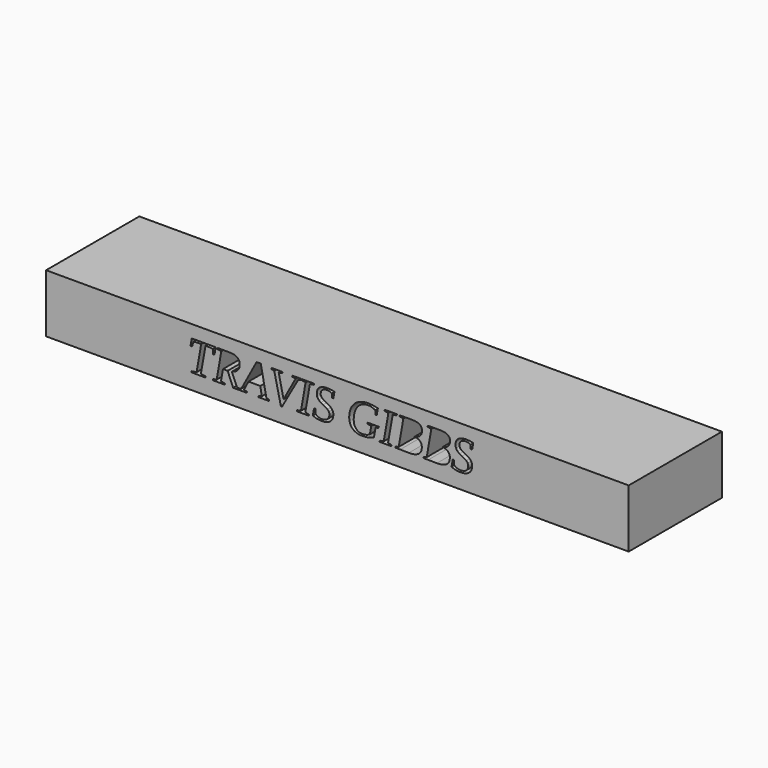
from build123d import *

# Parameters (mm, degrees)
F0_W     = 127
F0_H     = 12.7
F1_DEPTH = 25.4


with BuildPart() as f1:
    # F0 (on Front) → F1 (new body)
    with BuildSketch(Plane.XZ):
        with Locations((-1.1512227356, 52.6019901231)):
            Rectangle(F0_W, F0_H)
        with BuildLine():
            Line((-29.9385481048, 49.6464967728), (-32.9583853923, 49.6464967728))
            Line((-32.9583853923, 49.6464967728), (-32.9099805547, 49.9056968709))
            Line((-32.9099805547, 49.9056968709), (-31.8513199131, 50.0368583663))
            Line((-31.8513199131, 50.0368583663), (-30.8410641091, 55.7704894519))
            Line((-30.8410641091, 55.7704894519), (-31.0893340825, 55.7704894519))
            add(Edge.make_bspline(
                [(-31.0893340825, 55.7704894519), (-32.0605537272, 55.7704894519), (-32.5243033003, 55.6721183303)],
                knots=[0, 0, 0, 1, 1, 1], degree=2))
            Line((-32.5243033003, 55.6721183303), (-32.8365925751, 54.6524938481))
            Line((-32.8365925751, 54.6524938481), (-33.1629348673, 54.6524938481))
            Line((-33.1629348673, 54.6524938481), (-32.8896817518, 56.1905185265))
            Line((-32.8896817518, 56.1905185265), (-27.6682050769, 56.1905185265))
            Line((-27.6682050769, 56.1905185265), (-27.9414581924, 54.6524938481))
            Line((-27.9414581924, 54.6524938481), (-28.2740462701, 54.6524938481))
            Line((-28.2740462701, 54.6524938481), (-28.2256414325, 55.6721183303))
            add(Edge.make_bspline(
                [(-28.2256414325, 55.6721183303), (-28.6644078636, 55.7611207736), (-29.6590492039, 55.7611207736)],
                knots=[0, 0, 0, 1, 1, 1], degree=2))
            Line((-29.6590492039, 55.7611207736), (-29.8995119455, 55.7611207736))
            Line((-29.8995119455, 55.7611207736), (-30.9082063031, 50.0368583663))
            Line((-30.9082063031, 50.0368583663), (-29.8885818209, 49.9056968709))
            Line((-29.8885818209, 49.9056968709), (-29.9385481048, 49.6464967728))
        make_face(mode=Mode.SUBTRACT)
        with BuildLine():
            Line((-25.0730812032, 52.5164352083), (-26.0927056855, 52.5164352083))
            Line((-26.0927056855, 52.5164352083), (-26.533033563, 50.0368583663))
            Line((-26.533033563, 50.0368583663), (-25.6586235935, 49.9056968709))
            Line((-25.6586235935, 49.9056968709), (-25.7085898775, 49.6464967728))
            Line((-25.7085898775, 49.6464967728), (-28.3130824294, 49.6464967728))
            Line((-28.3130824294, 49.6464967728), (-28.2646775918, 49.9056968709))
            Line((-28.2646775918, 49.9056968709), (-27.4745857265, 50.0368583663))
            Line((-27.4745857265, 50.0368583663), (-26.4549612443, 55.8048412721))
            Line((-26.4549612443, 55.8048412721), (-27.2747205907, 55.9313184284))
            Line((-27.2747205907, 55.9313184284), (-27.2247543067, 56.1905185265))
            Line((-27.2247543067, 56.1905185265), (-24.629630433, 56.1905185265))
            add(Edge.make_bspline(
                [(-24.629630433, 56.1905185265), (-23.5616011131, 56.1905185265), (-23.0002611416, 55.7853231924)],
                knots=[0, 0, 0, 1, 1, 1], degree=2))
            add(Edge.make_bspline(
                [(-23.0002611416, 55.7853231924), (-22.4389211702, 55.3801278584), (-22.4389211702, 54.6040890105)],
                knots=[0, 0, 0, 1, 1, 1], degree=2))
            add(Edge.make_bspline(
                [(-22.4389211702, 54.6040890105), (-22.4389211702, 53.0629414392), (-24.1471435034, 52.6522810429)],
                knots=[0, 0, 0, 1, 1, 1], degree=2))
            Line((-24.1471435034, 52.6522810429), (-23.0385165778, 50.0368583663))
            Line((-23.0385165778, 50.0368583663), (-22.5105122318, 49.94023012))
            Line((-22.5105122318, 49.94023012), (-22.1078945389, 50.0368583663))
            Line((-22.1078945389, 50.0368583663), (-18.7788908693, 56.2436077032))
            Line((-18.7788908693, 56.2436077032), (-17.8482688304, 56.2436077032))
            Line((-17.8482688304, 56.2436077032), (-16.6272177658, 50.0368583663))
            Line((-16.6272177658, 50.0368583663), (-16.01825368, 49.9056968709))
            Line((-16.01825368, 49.9056968709), (-16.0713428567, 49.6464967728))
            Line((-16.0713428567, 49.6464967728), (-18.3885292758, 49.6464967728))
            Line((-18.3885292758, 49.6464967728), (-18.3354400991, 49.9056968709))
            Line((-18.3354400991, 49.9056968709), (-17.6374735699, 50.0368583663))
            Line((-17.6374735699, 50.0368583663), (-17.9497628447, 51.9246470325))
            Line((-17.9497628447, 51.9246470325), (-20.5261493619, 51.9246470325))
            Line((-20.5261493619, 51.9246470325), (-21.5270364877, 50.0368583663))
            Line((-21.5270364877, 50.0368583663), (-20.8681061178, 49.9056968709))
            Line((-20.8681061178, 49.9056968709), (-20.9165109554, 49.6464967728))
            Line((-20.9165109554, 49.6464967728), (-22.3702175297, 49.6464967728))
            Line((-22.3702175297, 49.6464967728), (-22.7028056074, 49.6464967728))
            Line((-22.7028056074, 49.6464967728), (-23.8738903879, 49.6464967728))
            Line((-23.8738903879, 49.6464967728), (-25.0730812032, 52.5164352083))
        make_face(mode=Mode.SUBTRACT)
        Polygon((-10.9529216425, 56.1905185265), (-8.9870606575, 56.1905185265), (-9.0354654951, 55.9313184284), (-9.6756585085, 55.8048412721), (-13.221703224, 49.4950364745), (-13.4715346438, 49.4950364745), (-14.9111882007, 55.8048412721), (-15.5310824112, 55.9313184284), (-15.4811161273, 56.1905185265), (-13.0764887112, 56.1905185265), (-13.1248935488, 55.9313184284), (-13.9493372343, 55.8048412721), (-12.8859922536, 51.0268153674), (-10.2658852379, 55.8048412721), (-11.0075722655, 55.9313184284), align=None, mode=Mode.SUBTRACT)
        Polygon((-7.1383081506, 55.8048412721), (-8.1485639546, 50.0368583663), (-7.3381732865, 49.9056968709), (-7.3772094458, 49.6464967728), (-9.9879477833, 49.6464967728), (-9.9489116239, 49.9056968709), (-9.0901161182, 50.0368583663), (-8.0798603142, 55.8048412721), (-8.8902509823, 55.9313184284), (-8.851214823, 56.1905185265), (-6.2311078073, 56.1905185265), (-6.2701439666, 55.9313184284), align=None, mode=Mode.SUBTRACT)
        with BuildLine():
            Line((-6.5043609227, 50.0025065461), (-6.2498451637, 51.4562131203))
            Line((-6.2498451637, 51.4562131203), (-5.9328715498, 51.4562131203))
            Line((-5.9328715498, 51.4562131203), (-5.9281872107, 50.5255910814))
            add(Edge.make_bspline(
                [(-5.9281872107, 50.5255910814), (-5.7673582342, 50.2804440006), (-5.3793388102, 50.1125885154)],
                knots=[0, 0, 0, 1, 1, 1], degree=2))
            add(Edge.make_bspline(
                [(-5.3793388102, 50.1125885154), (-4.9913193862, 49.9447330302), (-4.5572372942, 49.9447330302)],
                knots=[0, 0, 0, 1, 1, 1], degree=2))
            add(Edge.make_bspline(
                [(-4.5572372942, 49.9447330302), (-3.7577767507, 49.9447330302), (-3.3252561051, 50.3226030527)],
                knots=[0, 0, 0, 1, 1, 1], degree=2))
            add(Edge.make_bspline(
                [(-3.3252561051, 50.3226030527), (-2.8927354595, 50.7004730753), (-2.8927354595, 51.3781408016)],
                knots=[0, 0, 0, 1, 1, 1], degree=2))
            add(Edge.make_bspline(
                [(-2.8927354595, 51.3781408016), (-2.8927354595, 51.6420252388), (-3.0098439375, 51.8372060356)],
                knots=[0, 0, 0, 1, 1, 1], degree=2))
            add(Edge.make_bspline(
                [(-3.0098439375, 51.8372060356), (-3.1269524156, 52.0323868324), (-3.3221332124, 52.1885314698)],
                knots=[0, 0, 0, 1, 1, 1], degree=2))
            add(Edge.make_bspline(
                [(-3.3221332124, 52.1885314698), (-3.5173140091, 52.3446761072), (-3.7640225362, 52.4766183258)],
                knots=[0, 0, 0, 1, 1, 1], degree=2))
            add(Edge.make_bspline(
                [(-3.7640225362, 52.4766183258), (-4.0107310633, 52.6085605444), (-4.2691504382, 52.7428449326)],
                knots=[0, 0, 0, 1, 1, 1], degree=2))
            add(Edge.make_bspline(
                [(-4.2691504382, 52.7428449326), (-4.5275698131, 52.8771293207), (-4.7742783402, 53.0309317886)],
                knots=[0, 0, 0, 1, 1, 1], degree=2))
            add(Edge.make_bspline(
                [(-4.7742783402, 53.0309317886), (-5.0209868673, 53.1847342564), (-5.2161676641, 53.3869415619)],
                knots=[0, 0, 0, 1, 1, 1], degree=2))
            add(Edge.make_bspline(
                [(-5.2161676641, 53.3869415619), (-5.4113484609, 53.5891488673), (-5.5284569389, 53.8530333045)],
                knots=[0, 0, 0, 1, 1, 1], degree=2))
            add(Edge.make_bspline(
                [(-5.5284569389, 53.8530333045), (-5.645565417, 54.1169177417), (-5.645565417, 54.472927515)],
                knots=[0, 0, 0, 1, 1, 1], degree=2))
            add(Edge.make_bspline(
                [(-5.645565417, 54.472927515), (-5.645565417, 55.341091699), (-5.0553386876, 55.8024991026)],
                knots=[0, 0, 0, 1, 1, 1], degree=2))
            add(Edge.make_bspline(
                [(-5.0553386876, 55.8024991026), (-4.4651119582, 56.2639065061), (-3.3674151572, 56.2639065061)],
                knots=[0, 0, 0, 1, 1, 1], degree=2))
            add(Edge.make_bspline(
                [(-3.3674151572, 56.2639065061), (-2.5273570079, 56.2639065061), (-1.7856699803, 56.0780943876)],
                knots=[0, 0, 0, 1, 1, 1], degree=2))
            Line((-1.7856699803, 56.0780943876), (-2.0245712755, 54.7165131494))
            Line((-2.0245712755, 54.7165131494), (-2.3415448894, 54.7165131494))
            Line((-2.3415448894, 54.7165131494), (-2.3665280314, 55.5503255131))
            add(Edge.make_bspline(
                [(-2.3665280314, 55.5503255131), (-2.5226726688, 55.6783641158), (-2.8006101234, 55.7658051128)],
                knots=[0, 0, 0, 1, 1, 1], degree=2))
            add(Edge.make_bspline(
                [(-2.8006101234, 55.7658051128), (-3.078547578, 55.8532461097), (-3.4392416904, 55.8532461097)],
                knots=[0, 0, 0, 1, 1, 1], degree=2))
            add(Edge.make_bspline(
                [(-3.4392416904, 55.8532461097), (-4.088803382, 55.8532461097), (-4.4401288162, 55.5362724958)],
                knots=[0, 0, 0, 1, 1, 1], degree=2))
            add(Edge.make_bspline(
                [(-4.4401288162, 55.5362724958), (-4.7914542504, 55.2192988818), (-4.7914542504, 54.6478095089)],
                knots=[0, 0, 0, 1, 1, 1], degree=2))
            add(Edge.make_bspline(
                [(-4.7914542504, 54.6478095089), (-4.7914542504, 54.3402045732), (-4.5720710348, 54.0864695374)],
                knots=[0, 0, 0, 1, 1, 1], degree=2))
            add(Edge.make_bspline(
                [(-4.5720710348, 54.0864695374), (-4.3526878192, 53.8327345017), (-3.9186057272, 53.6141320093)],
                knots=[0, 0, 0, 1, 1, 1], degree=2))
            add(Edge.make_bspline(
                [(-3.9186057272, 53.6141320093), (-3.2549910183, 53.2674909142), (-2.9622198231, 53.087143858)],
                knots=[0, 0, 0, 1, 1, 1], degree=2))
            add(Edge.make_bspline(
                [(-2.9622198231, 53.087143858), (-2.669448628, 52.9067968018), (-2.4719256617, 52.7014666036)],
                knots=[0, 0, 0, 1, 1, 1], degree=2))
            add(Edge.make_bspline(
                [(-2.4719256617, 52.7014666036), (-2.2744026953, 52.4961364055), (-2.1541713245, 52.2330326914)],
                knots=[0, 0, 0, 1, 1, 1], degree=2))
            add(Edge.make_bspline(
                [(-2.1541713245, 52.2330326914), (-2.0339399537, 51.9699289774), (-2.0339399537, 51.6279722215)],
                knots=[0, 0, 0, 1, 1, 1], degree=2))
            add(Edge.make_bspline(
                [(-2.0339399537, 51.6279722215), (-2.0339399537, 50.6224007566), (-2.690528154, 50.0852632039)],
                knots=[0, 0, 0, 1, 1, 1], degree=2))
            add(Edge.make_bspline(
                [(-2.690528154, 50.0852632039), (-3.3471163543, 49.5481256512), (-4.5869047754, 49.5481256512)],
                knots=[0, 0, 0, 1, 1, 1], degree=2))
            add(Edge.make_bspline(
                [(-4.5869047754, 49.5481256512), (-5.2021146467, 49.5481256512), (-5.6924088082, 49.6730413611)],
                knots=[0, 0, 0, 1, 1, 1], degree=2))
            add(Edge.make_bspline(
                [(-5.6924088082, 49.6730413611), (-6.1827029697, 49.7979570711), (-6.5043609227, 50.0025065461)],
                knots=[0, 0, 0, 1, 1, 1], degree=2))
        make_face(mode=Mode.SUBTRACT)
        with BuildLine():
            add(Edge.make_bspline(
                [(5.4703713201, 49.6714799148), (4.8754602515, 49.5590557758), (4.2399515773, 49.5590557758)],
                knots=[0, 0, 0, 1, 1, 1], degree=2))
            add(Edge.make_bspline(
                [(4.2399515773, 49.5590557758), (2.9080378202, 49.5590557758), (2.1663507925, 50.2593644746)],
                knots=[0, 0, 0, 1, 1, 1], degree=2))
            add(Edge.make_bspline(
                [(2.1663507925, 50.2593644746), (1.4246637648, 50.9596731734), (1.4246637648, 52.197900148)],
                knots=[0, 0, 0, 1, 1, 1], degree=2))
            add(Edge.make_bspline(
                [(1.4246637648, 52.197900148), (1.4246637648, 53.4236355517), (1.9321338364, 54.3456696355)],
                knots=[0, 0, 0, 1, 1, 1], degree=2))
            add(Edge.make_bspline(
                [(1.9321338364, 54.3456696355), (2.439603908, 55.2677037194), (3.3671030542, 55.7658051128)],
                knots=[0, 0, 0, 1, 1, 1], degree=2))
            add(Edge.make_bspline(
                [(3.3671030542, 55.7658051128), (4.2946022004, 56.2639065061), (5.4937930157, 56.2639065061)],
                knots=[0, 0, 0, 1, 1, 1], degree=2))
            add(Edge.make_bspline(
                [(5.4937930157, 56.2639065061), (6.6211572978, 56.2639065061), (7.6751336003, 55.9703545878)],
                knots=[0, 0, 0, 1, 1, 1], degree=2))
            Line((7.6751336003, 55.9703545878), (7.4268636268, 54.5650528511))
            Line((7.4268636268, 54.5650528511), (7.1005213346, 54.5650528511))
            Line((7.1005213346, 54.5650528511), (7.114574352, 55.3754435192))
            add(Edge.make_bspline(
                [(7.114574352, 55.3754435192), (6.4946801415, 55.8735449126), (5.4656869809, 55.8735449126)],
                knots=[0, 0, 0, 1, 1, 1], degree=2))
            add(Edge.make_bspline(
                [(5.4656869809, 55.8735449126), (4.6022071361, 55.8735449126), (3.8995562677, 55.4074531699)],
                knots=[0, 0, 0, 1, 1, 1], degree=2))
            add(Edge.make_bspline(
                [(3.8995562677, 55.4074531699), (3.1969053994, 54.9413614273), (2.8010787436, 54.0825659215)],
                knots=[0, 0, 0, 1, 1, 1], degree=2))
            add(Edge.make_bspline(
                [(2.8010787436, 54.0825659215), (2.4052520878, 53.2237704158), (2.4052520878, 52.1010904728)],
                knots=[0, 0, 0, 1, 1, 1], degree=2))
            add(Edge.make_bspline(
                [(2.4052520878, 52.1010904728), (2.4052520878, 51.0861503297), (2.9056956506, 50.5177838495)],
                knots=[0, 0, 0, 1, 1, 1], degree=2))
            add(Edge.make_bspline(
                [(2.9056956506, 50.5177838495), (3.4061392135, 49.9494173693), (4.3039708786, 49.9494173693)],
                knots=[0, 0, 0, 1, 1, 1], degree=2))
            add(Edge.make_bspline(
                [(4.3039708786, 49.9494173693), (4.7380529706, 49.9494173693), (5.1776001249, 50.0735523561)],
                knots=[0, 0, 0, 1, 1, 1], degree=2))
            add(Edge.make_bspline(
                [(5.1776001249, 50.0735523561), (5.6171472792, 50.1976873428), (5.9231907685, 50.3928681396)],
                knots=[0, 0, 0, 1, 1, 1], degree=2))
            Line((5.9231907685, 50.3928681396), (6.2307957042, 52.1151434902))
            Line((6.2307957042, 52.1151434902), (5.415720697, 52.2431820929))
            Line((5.415720697, 52.2431820929), (5.4610026418, 52.5055050837))
            Line((5.4610026418, 52.5055050837), (7.8749987361, 52.5055050837))
            Line((7.8749987361, 52.5055050837), (7.8312782377, 52.2431820929))
            Line((7.8312782377, 52.2431820929), (7.1676635287, 52.1151434902))
            Line((7.1676635287, 52.1151434902), (6.8022850772, 50.0665258474))
            add(Edge.make_bspline(
                [(6.8022850772, 50.0665258474), (6.0652823886, 49.7839040537), (5.4703713201, 49.6714799148)],
                knots=[0, 0, 0, 1, 1, 1], degree=2))
        make_face(mode=Mode.SUBTRACT)
        Polygon((10.9010818091, 55.8048412721), (9.8908260051, 50.0368583663), (10.7012166732, 49.9056968709), (10.6621805139, 49.6464967728), (8.0514421764, 49.6464967728), (8.0904783358, 49.9056968709), (8.9492738415, 50.0368583663), (9.9595296455, 55.8048412721), (9.1491389774, 55.9313184284), (9.1881751367, 56.1905185265), (11.8082821524, 56.1905185265), (11.7692459931, 55.9313184284), align=None, mode=Mode.SUBTRACT)
        with BuildLine():
            Line((12.5499691801, 49.6464967728), (11.510045895, 49.6464967728))
            Line((11.510045895, 49.6464967728), (11.560012179, 49.9056968709))
            Line((11.560012179, 49.9056968709), (12.2080124242, 50.0368583663))
            Line((12.2080124242, 50.0368583663), (13.2276369065, 55.8048412721))
            Line((13.2276369065, 55.8048412721), (12.4078775601, 55.9313184284))
            Line((12.4078775601, 55.9313184284), (12.4578438441, 56.1905185265))
            Line((12.4578438441, 56.1905185265), (15.1466545002, 56.1905185265))
            add(Edge.make_bspline(
                [(15.1466545002, 56.1905185265), (17.3030119428, 56.1905185265), (17.3030119428, 54.8133228246)],
                knots=[0, 0, 0, 1, 1, 1], degree=2))
            add(Edge.make_bspline(
                [(17.3030119428, 54.8133228246), (17.3030119428, 54.12628642), (16.8712720204, 53.6773705874)],
                knots=[0, 0, 0, 1, 1, 1], degree=2))
            add(Edge.make_bspline(
                [(16.8712720204, 53.6773705874), (16.4395320979, 53.2284547549), (15.6681775892, 53.1253992942)],
                knots=[0, 0, 0, 1, 1, 1], degree=2))
            add(Edge.make_bspline(
                [(15.6681775892, 53.1253992942), (16.4239176342, 53.0629414392), (16.8392623697, 52.6749220153)],
                knots=[0, 0, 0, 1, 1, 1], degree=2))
            add(Edge.make_bspline(
                [(16.8392623697, 52.6749220153), (17.2546071052, 52.2869025913), (17.2546071052, 51.646709578)],
                knots=[0, 0, 0, 1, 1, 1], degree=2))
            add(Edge.make_bspline(
                [(17.2546071052, 51.646709578), (17.2546071052, 50.5974176146), (16.544149005, 50.1071234531)],
                knots=[0, 0, 0, 1, 1, 1], degree=2))
            add(Edge.make_bspline(
                [(16.544149005, 50.1071234531), (15.8336909048, 49.6168292917), (14.4190204899, 49.6168292917)],
                knots=[0, 0, 0, 1, 1, 1], degree=2))
            Line((14.4190204899, 49.6168292917), (12.5499691801, 49.6464967728))
        make_face(mode=Mode.SUBTRACT)
        with BuildLine():
            Line((18.6536630564, 49.6464967728), (17.6137397713, 49.6464967728))
            Line((17.6137397713, 49.6464967728), (17.6637060552, 49.9056968709))
            Line((17.6637060552, 49.9056968709), (18.3117063005, 50.0368583663))
            Line((18.3117063005, 50.0368583663), (19.3313307827, 55.8048412721))
            Line((19.3313307827, 55.8048412721), (18.5115714363, 55.9313184284))
            Line((18.5115714363, 55.9313184284), (18.5615377203, 56.1905185265))
            Line((18.5615377203, 56.1905185265), (21.2503483765, 56.1905185265))
            add(Edge.make_bspline(
                [(21.2503483765, 56.1905185265), (23.4067058191, 56.1905185265), (23.4067058191, 54.8133228246)],
                knots=[0, 0, 0, 1, 1, 1], degree=2))
            add(Edge.make_bspline(
                [(23.4067058191, 54.8133228246), (23.4067058191, 54.12628642), (22.9749658966, 53.6773705874)],
                knots=[0, 0, 0, 1, 1, 1], degree=2))
            add(Edge.make_bspline(
                [(22.9749658966, 53.6773705874), (22.5432259742, 53.2284547549), (21.7718714654, 53.1253992942)],
                knots=[0, 0, 0, 1, 1, 1], degree=2))
            add(Edge.make_bspline(
                [(21.7718714654, 53.1253992942), (22.5276115105, 53.0629414392), (22.942956246, 52.6749220153)],
                knots=[0, 0, 0, 1, 1, 1], degree=2))
            add(Edge.make_bspline(
                [(22.942956246, 52.6749220153), (23.3583009815, 52.2869025913), (23.3583009815, 51.646709578)],
                knots=[0, 0, 0, 1, 1, 1], degree=2))
            add(Edge.make_bspline(
                [(23.3583009815, 51.646709578), (23.3583009815, 50.5974176146), (22.6478428813, 50.1071234531)],
                knots=[0, 0, 0, 1, 1, 1], degree=2))
            add(Edge.make_bspline(
                [(22.6478428813, 50.1071234531), (21.9373847811, 49.6168292917), (20.5227143662, 49.6168292917)],
                knots=[0, 0, 0, 1, 1, 1], degree=2))
            Line((20.5227143662, 49.6168292917), (18.6536630564, 49.6464967728))
        make_face(mode=Mode.SUBTRACT)
        with BuildLine():
            Line((23.7424167895, 50.0025065461), (23.9969325485, 51.4562131203))
            Line((23.9969325485, 51.4562131203), (24.3139061624, 51.4562131203))
            Line((24.3139061624, 51.4562131203), (24.3185905015, 50.5255910814))
            add(Edge.make_bspline(
                [(24.3185905015, 50.5255910814), (24.4794194781, 50.2804440006), (24.867438902, 50.1125885154)],
                knots=[0, 0, 0, 1, 1, 1], degree=2))
            add(Edge.make_bspline(
                [(24.867438902, 50.1125885154), (25.255458326, 49.9447330302), (25.689540418, 49.9447330302)],
                knots=[0, 0, 0, 1, 1, 1], degree=2))
            add(Edge.make_bspline(
                [(25.689540418, 49.9447330302), (26.4890009615, 49.9447330302), (26.9215216071, 50.3226030527)],
                knots=[0, 0, 0, 1, 1, 1], degree=2))
            add(Edge.make_bspline(
                [(26.9215216071, 50.3226030527), (27.3540422527, 50.7004730753), (27.3540422527, 51.3781408016)],
                knots=[0, 0, 0, 1, 1, 1], degree=2))
            add(Edge.make_bspline(
                [(27.3540422527, 51.3781408016), (27.3540422527, 51.6420252388), (27.2369337747, 51.8372060356)],
                knots=[0, 0, 0, 1, 1, 1], degree=2))
            add(Edge.make_bspline(
                [(27.2369337747, 51.8372060356), (27.1198252966, 52.0323868324), (26.9246444999, 52.1885314698)],
                knots=[0, 0, 0, 1, 1, 1], degree=2))
            add(Edge.make_bspline(
                [(26.9246444999, 52.1885314698), (26.7294637031, 52.3446761072), (26.482755176, 52.4766183258)],
                knots=[0, 0, 0, 1, 1, 1], degree=2))
            add(Edge.make_bspline(
                [(26.482755176, 52.4766183258), (26.2360466489, 52.6085605444), (25.977627274, 52.7428449326)],
                knots=[0, 0, 0, 1, 1, 1], degree=2))
            add(Edge.make_bspline(
                [(25.977627274, 52.7428449326), (25.7192078991, 52.8771293207), (25.472499372, 53.0309317886)],
                knots=[0, 0, 0, 1, 1, 1], degree=2))
            add(Edge.make_bspline(
                [(25.472499372, 53.0309317886), (25.2257908449, 53.1847342564), (25.0306100481, 53.3869415619)],
                knots=[0, 0, 0, 1, 1, 1], degree=2))
            add(Edge.make_bspline(
                [(25.0306100481, 53.3869415619), (24.8354292513, 53.5891488673), (24.7183207733, 53.8530333045)],
                knots=[0, 0, 0, 1, 1, 1], degree=2))
            add(Edge.make_bspline(
                [(24.7183207733, 53.8530333045), (24.6012122952, 54.1169177417), (24.6012122952, 54.472927515)],
                knots=[0, 0, 0, 1, 1, 1], degree=2))
            add(Edge.make_bspline(
                [(24.6012122952, 54.472927515), (24.6012122952, 55.341091699), (25.1914390246, 55.8024991026)],
                knots=[0, 0, 0, 1, 1, 1], degree=2))
            add(Edge.make_bspline(
                [(25.1914390246, 55.8024991026), (25.781665754, 56.2639065061), (26.879362555, 56.2639065061)],
                knots=[0, 0, 0, 1, 1, 1], degree=2))
            add(Edge.make_bspline(
                [(26.879362555, 56.2639065061), (27.7194207043, 56.2639065061), (28.461107732, 56.0780943876)],
                knots=[0, 0, 0, 1, 1, 1], degree=2))
            Line((28.461107732, 56.0780943876), (28.2222064367, 54.7165131494))
            Line((28.2222064367, 54.7165131494), (27.9052328228, 54.7165131494))
            Line((27.9052328228, 54.7165131494), (27.8802496808, 55.5503255131))
            add(Edge.make_bspline(
                [(27.8802496808, 55.5503255131), (27.7241050434, 55.6783641158), (27.4461675888, 55.7658051128)],
                knots=[0, 0, 0, 1, 1, 1], degree=2))
            add(Edge.make_bspline(
                [(27.4461675888, 55.7658051128), (27.1682301342, 55.8532461097), (26.8075360218, 55.8532461097)],
                knots=[0, 0, 0, 1, 1, 1], degree=2))
            add(Edge.make_bspline(
                [(26.8075360218, 55.8532461097), (26.1579743302, 55.8532461097), (25.806648896, 55.5362724958)],
                knots=[0, 0, 0, 1, 1, 1], degree=2))
            add(Edge.make_bspline(
                [(25.806648896, 55.5362724958), (25.4553234619, 55.2192988818), (25.4553234619, 54.6478095089)],
                knots=[0, 0, 0, 1, 1, 1], degree=2))
            add(Edge.make_bspline(
                [(25.4553234619, 54.6478095089), (25.4553234619, 54.3402045732), (25.6747066774, 54.0864695374)],
                knots=[0, 0, 0, 1, 1, 1], degree=2))
            add(Edge.make_bspline(
                [(25.6747066774, 54.0864695374), (25.894089893, 53.8327345017), (26.328171985, 53.6141320093)],
                knots=[0, 0, 0, 1, 1, 1], degree=2))
            add(Edge.make_bspline(
                [(26.328171985, 53.6141320093), (26.9917866939, 53.2674909142), (27.2845578891, 53.087143858)],
                knots=[0, 0, 0, 1, 1, 1], degree=2))
            add(Edge.make_bspline(
                [(27.2845578891, 53.087143858), (27.5773290842, 52.9067968018), (27.7748520505, 52.7014666036)],
                knots=[0, 0, 0, 1, 1, 1], degree=2))
            add(Edge.make_bspline(
                [(27.7748520505, 52.7014666036), (27.9723750169, 52.4961364055), (28.0926063877, 52.2330326914)],
                knots=[0, 0, 0, 1, 1, 1], degree=2))
            add(Edge.make_bspline(
                [(28.0926063877, 52.2330326914), (28.2128377585, 51.9699289774), (28.2128377585, 51.6279722215)],
                knots=[0, 0, 0, 1, 1, 1], degree=2))
            add(Edge.make_bspline(
                [(28.2128377585, 51.6279722215), (28.2128377585, 50.6224007566), (27.5562495582, 50.0852632039)],
                knots=[0, 0, 0, 1, 1, 1], degree=2))
            add(Edge.make_bspline(
                [(27.5562495582, 50.0852632039), (26.8996613579, 49.5481256512), (25.6598729369, 49.5481256512)],
                knots=[0, 0, 0, 1, 1, 1], degree=2))
            add(Edge.make_bspline(
                [(25.6598729369, 49.5481256512), (25.0446630655, 49.5481256512), (24.554368904, 49.6730413611)],
                knots=[0, 0, 0, 1, 1, 1], degree=2))
            add(Edge.make_bspline(
                [(24.554368904, 49.6730413611), (24.0640747426, 49.7979570711), (23.7424167895, 50.0025065461)],
                knots=[0, 0, 0, 1, 1, 1], degree=2))
        make_face(mode=Mode.SUBTRACT)
    extrude(amount=F1_DEPTH)


solid = f1.part
